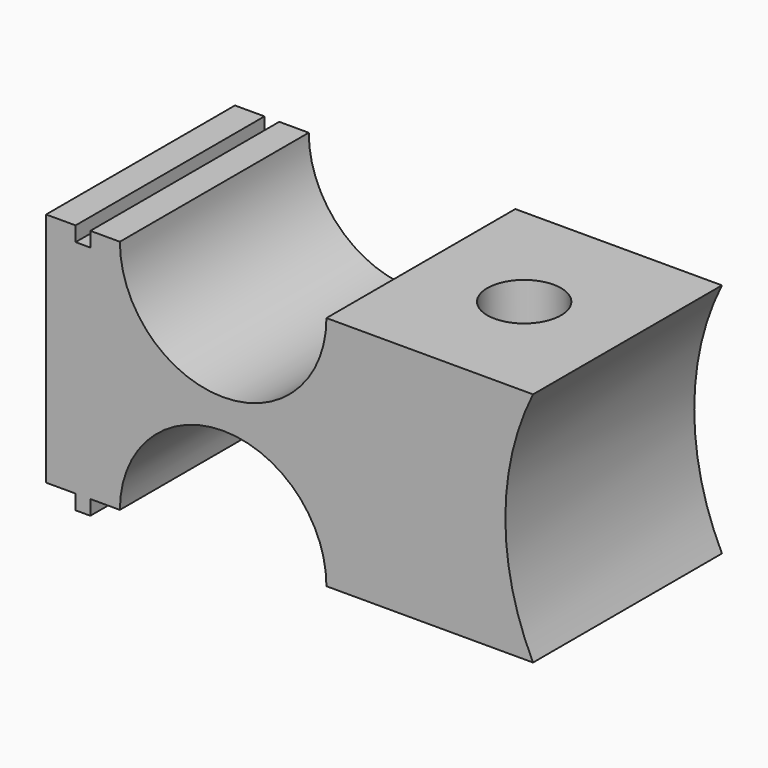
from build123d import *

# Parameters (mm, degrees)
F1_DEPTH = 16
F3_D     = 5
F4_W     = 1
F4_H     = 16
F5_DEPTH = 1
F6_W     = 1
F6_H     = 16
F7_DEPTH = 1


# Not quite as in the source:
# - a feature names something its author has since deleted; it is built from what else it names


with BuildPart() as f1:
    # F0 (on Front) → F1 (new body)
    with BuildSketch(Plane.XZ):
        with BuildLine():
            Line((-21, 8), (-21, -8))
            Line((-21, -8), (-16, -8))
            ThreePointArc((-16, -8), (-9, -1), (-2, -8))
            Line((-2, -8), (12.0004845034, -8))
            ThreePointArc((12.0004845034, -8), (10.125, 0), (12.0004845034, 8))
            Line((12.0004845034, 8), (-2, 8))
            ThreePointArc((-2, 8), (-9, 1), (-16, 8))
            Line((-16, 8), (-21, 8))
        make_face()
    extrude(amount=F1_DEPTH)

    # F3 (through all)
    with Locations(Plane.XY.offset(8)):
        with Locations((5, -8)):
            Hole(F3_D / 2)

    # F4 (on face) → F5 (cut)
    with BuildSketch(Plane.XY.offset(8)):
        with Locations((-18.5, -8)):
            Rectangle(F4_W, F4_H)
    extrude(amount=-F5_DEPTH, mode=Mode.SUBTRACT)

    # F6 (on face) → F7 (join)
    with BuildSketch(Plane(origin=(0, 0, -8), x_dir=(1, 0, 0), z_dir=(0, 0, -1))):
        with Locations((-18.5, 8)):
            Rectangle(F6_W, F6_H)
    extrude(amount=F7_DEPTH)


solid = f1.part
